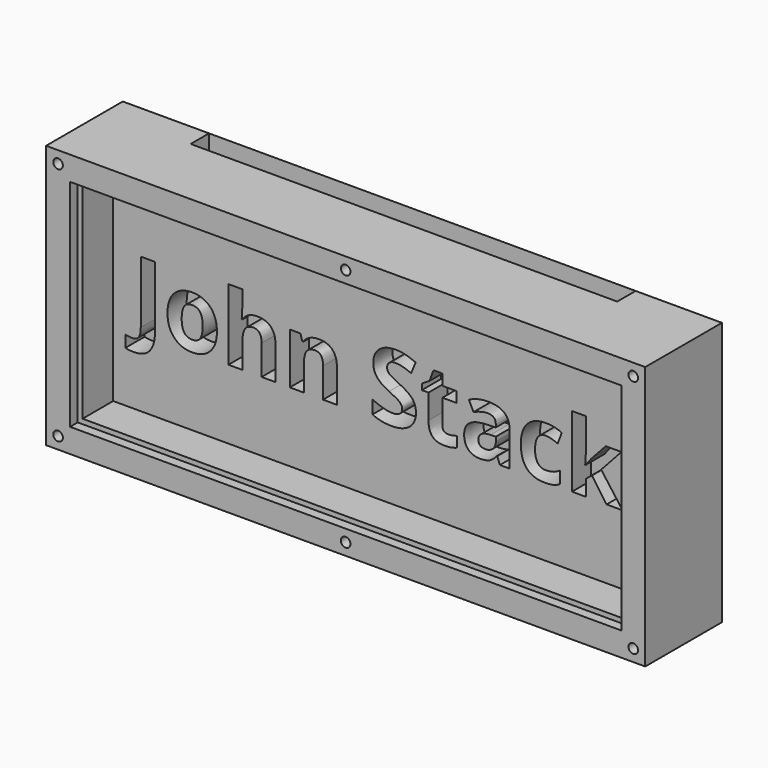
from build123d import *

# Parameters (mm, degrees)
F0_W          = 125
F0_H          = 55
F1_DEPTH      = 11
F2_W          = 125
F2_H          = 55
F2_W_2        = 113
F2_H_2        = 43
F3_DEPTH      = 8
F4_W          = 125
F4_H          = 55
F4_W_2        = 115
F4_H_2        = 45
F5_DEPTH      = 2
F6_R          = 1
F7_DEPTH      = 2.5
F8_TEXT_SIZE  = 9.1515729266
F9_DEPTH      = 1
F10_TEXT_SIZE = 19.4918194444
F11_DEPTH     = 5
F12_SIZE      = 1
F14_DEPTH     = 20


# Not quite as in the source:
# - Text() gives the source's letters only with a copy of the font that has no kerning and outlines rounded to 1/6400 em; it was checked with that copy


with BuildPart() as f1:
    # F0 (on Front) → F1 (new body)
    with BuildSketch(Plane.XZ):
        with Locations((62.5, 27.5)):
            Rectangle(F0_W, F0_H)
    extrude(amount=F1_DEPTH)

    # F2 (on face) → F3 (join)
    with BuildSketch(Plane.XZ.offset(11)):
        with Locations((62.5, 27.5)):
            Rectangle(F2_W, F2_H)
        with Locations((62.5, 27.5)):
            Rectangle(F2_W_2, F2_H_2, mode=Mode.SUBTRACT)
    extrude(amount=F3_DEPTH)

    # F4 (on face) → F5 (join)
    with BuildSketch(Plane.XZ.offset(19)):
        with Locations((62.5, 27.5)):
            Rectangle(F4_W, F4_H)
        with Locations((62.5, 27.5)):
            Rectangle(F4_W_2, F4_H_2, mode=Mode.SUBTRACT)
    extrude(amount=F5_DEPTH)

    # F6 (on face) → F7 (cut)
    with BuildSketch(Plane.XZ.offset(21)):
        with Locations((122.5, 52.5)):
            Circle(F6_R)
        with Locations((122.5, 2.5)):
            Circle(F6_R)
        with Locations((62.5, 2.5)):
            Circle(F6_R)
        with Locations((62.5, 52.5)):
            Circle(F6_R)
        with Locations((2.5, 52.5)):
            Circle(F6_R)
        with Locations((2.5, 2.5)):
            Circle(F6_R)
    extrude(amount=-F7_DEPTH, mode=Mode.SUBTRACT)

    # F8 (on face) → F9 (cut)
    with BuildSketch(Plane(origin=(0, 0, 0), x_dir=(-1, 0, 0), z_dir=(0, 1, 0))):
        with Locations((-32, 2)):
            Text('Cashel', F8_TEXT_SIZE, font='Open Sans', font_style=FontStyle.BOLD, text_align=(TextAlign.LEFT, TextAlign.BOTTOM))
    extrude(amount=-F9_DEPTH, mode=Mode.SUBTRACT)

    # F10 (on face) → F11 (cut)
    with BuildSketch(Plane.XZ.offset(11)):
        with Locations((10.0000051302, 20.482945)):
            Text('John Stack', F10_TEXT_SIZE, font='Open Sans', font_style=FontStyle.BOLD, text_align=(TextAlign.LEFT, TextAlign.BOTTOM))
    extrude(amount=-F11_DEPTH, mode=Mode.SUBTRACT)

    # F12
    f12_edges = [f1.edges().sort_by_distance(p)[0] for p in [
        (62.5, 0, 55),
        (125, 0, 27.5),
        (62.5, 0, 0),
        (0, 0, 27.5),
    ]]
    chamfer(f12_edges, length=F12_SIZE)

    # F13 (on face) → F14 (cut)
    with BuildSketch(Plane.XY.offset(55)):
        Polygon((107, -1), (62.5, -1), (18, -1), (18, -5.8), (107, -5.8), align=None)
    extrude(amount=-F14_DEPTH, mode=Mode.SUBTRACT)


solid = f1.part
